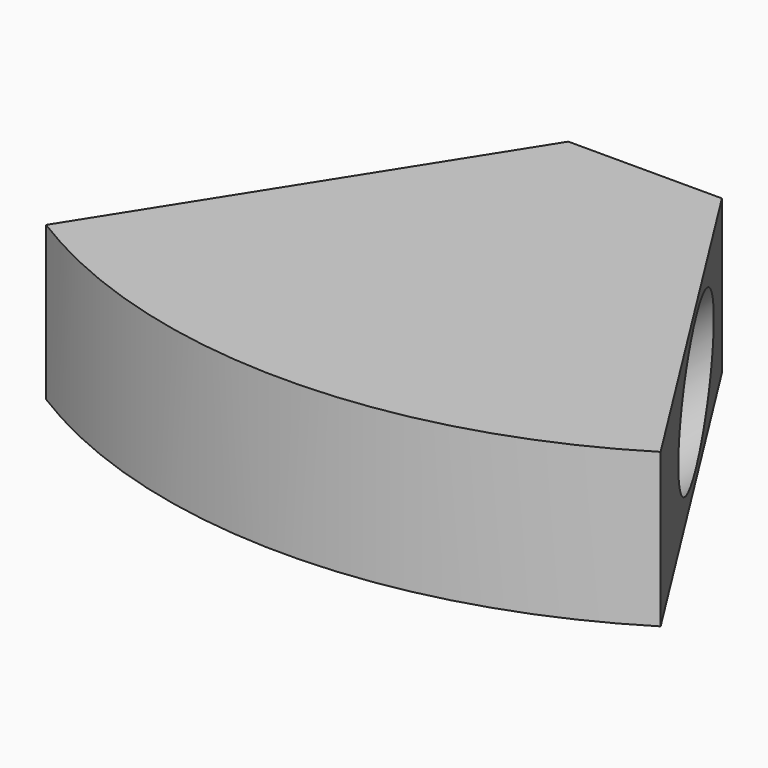
from build123d import *

# Parameters (mm, degrees)
F1_DEPTH = 30
F3_R     = 13
F3_R_2   = 11
F4_DEPTH = 75


# Not quite as in the source:
# - the program builds the solid bodies; features that only make, move or delete a surface that nothing else refers to are left out


with BuildPart() as f1:
    # F0 (on Top) → F1 (new body)
    with BuildSketch(Plane.XY):
        with BuildLine():
            Line((0, 0), (-15, 0))
            Line((-15, 0), (-60, -71.2145941459))
            ThreePointArc((-60, -71.2145941459), (0, -88.4018294902), (60, -71.2145941459))
            Line((60, -71.2145941459), (15, 0))
            Line((15, 0), (0, 0))
        make_face()
    extrude(amount=F1_DEPTH)

    # F3 (on Front) → F4 (cut)
    with BuildSketch(Plane.XZ):
        with Locations((-34, 15.2476818305)):
            Circle(F3_R)
        with Locations((-34, 15.2476818305)):
            Circle(F3_R_2, mode=Mode.SUBTRACT)
        with Locations((0, 15.1581136116)):
            Circle(F3_R)
        with Locations((0, 15.1581136116)):
            Circle(F3_R_2, mode=Mode.SUBTRACT)
        with Locations((34, 15.0685453927)):
            Circle(F3_R)
        with Locations((34, 15.0685453927)):
            Circle(F3_R_2, mode=Mode.SUBTRACT)
        with Locations((0, 15.1581136116)):
            Circle(F3_R_2)
        with Locations((34, 15.0685453927)):
            Circle(F3_R_2)
        with Locations((-34, 15.2476818305)):
            Circle(F3_R_2)
    extrude(amount=F4_DEPTH, mode=Mode.SUBTRACT)


solid = f1.part
